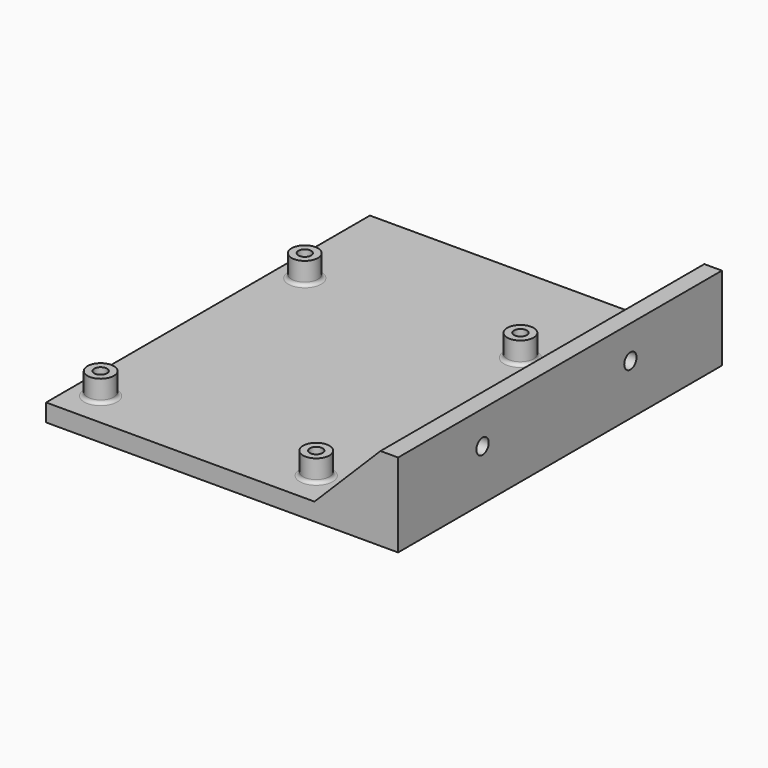
from build123d import *

# Parameters (mm, degrees)
F0_W      = 80
F0_H      = 92
F1_DEPTH  = 4
F3_R      = 3
F4_DEPTH  = 5
F6_R      = 1.45
F7_DEPTH  = 8.5
F8_R      = 0.75
F9_W      = 4
F9_H      = 92
F10_DEPTH = 15
F11_R     = 1.75
F12_DEPTH = 4
F14_DEPTH = 4
F16_DEPTH = 4


with BuildPart() as f1:
    # F0 (on Top) → F1 (new body)
    with BuildSketch(Plane.XY):
        Rectangle(F0_W, F0_H)
    extrude(amount=-F1_DEPTH)

    # F3 (on face) → F4 (join)
    with BuildSketch(Plane.XY):
        with Locations((-34, 20)):
            Circle(F3_R)
        with Locations((15, 20)):
            Circle(F3_R)
        with Locations((15, -38)):
            Circle(F3_R)
        with Locations((-34, -38)):
            Circle(F3_R)
    extrude(amount=F4_DEPTH)

    # F6 (on face) → F7 (cut, through all)
    with BuildSketch(Plane.XY.offset(5)):
        with Locations((-34, 20)):
            Circle(F6_R)
        with Locations((15, 20)):
            Circle(F6_R)
        with Locations((15, -38)):
            Circle(F6_R)
        with Locations((-34, -38)):
            Circle(F6_R)
    extrude(amount=-F7_DEPTH, mode=Mode.SUBTRACT)

    # F8
    f8_edges = [f1.edges().sort_by_distance(p)[0] for p in [
        (12, -38, 0),
        (-37, -38, 0),
        (12, 20, 0),
        (-37, 20, 0),
        (13.55, -38, -3.5),
        (-35.45, -38, -3.5),
        (-35.45, 20, -3.5),
        (13.55, 20, -3.5),
    ]]
    fillet(f8_edges, radius=F8_R)

    # F9 (on face) → F10 (join)
    with BuildSketch(Plane.XY):
        with Locations((38, 0)):
            Rectangle(F9_W, F9_H)
    extrude(amount=F10_DEPTH)

    # F11 (on face) → F12 (cut, through all)
    with BuildSketch(Plane(origin=(36, 0, 0), x_dir=(0, -1, 0), z_dir=(-1, 0, 0))):
        with Locations((-20, 7.5)):
            Circle(F11_R)
        with Locations((22, 7.5)):
            Circle(F11_R)
    extrude(amount=-F12_DEPTH, mode=Mode.SUBTRACT)

    # F13 (on face) → F14 (join)
    with BuildSketch(Plane(origin=(0, 46, 0), x_dir=(-1, 0, 0), z_dir=(0, 1, 0))):
        Polygon((-21, 0), (-36, 15), (-36, 0), align=None)
    extrude(amount=-F14_DEPTH)

    # F15 (on face) → F16 (join)
    with BuildSketch(Plane.XZ.offset(46)):
        Polygon((36, 0), (36, 15), (21, 0), align=None)
    extrude(amount=-F16_DEPTH)


solid = f1.part
